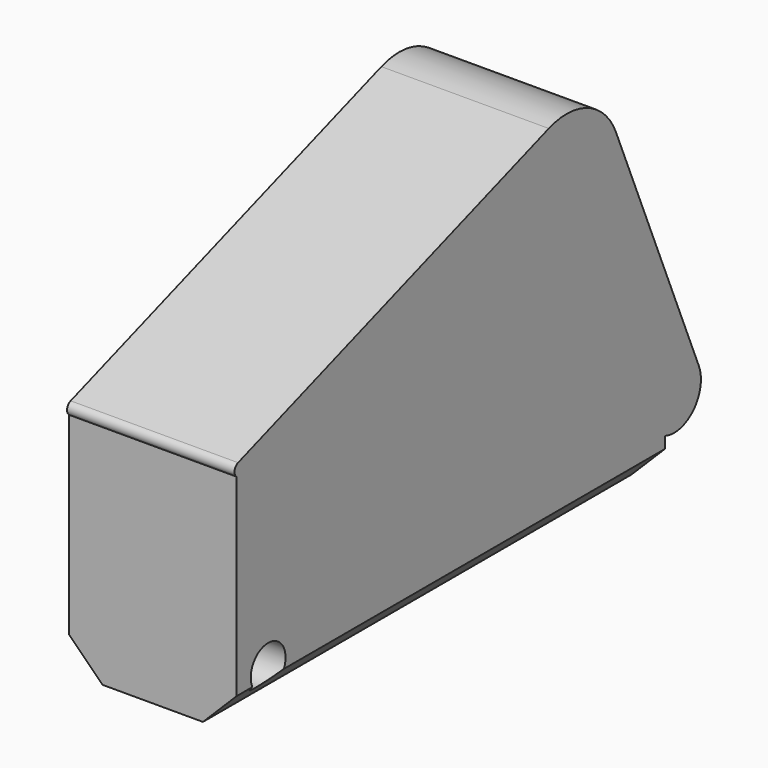
from build123d import *

# Parameters (mm, degrees)
F1_DEPTH     = 25
F3_DEPTH     = 25
F5_D         = 6.5
F6_R         = 10
F7_R         = 5
F8_T1_DEPTH  = 38.943500224
F9_T1_DEPTH  = 105.7168298797
F10_T1_DEPTH = 105.7168298797


# Not quite as in the source:
# - a fillet or chamfer that OpenCascade refuses, or shapes differently, is made with other operations: its cross-section is extruded or revolved along the edge and cut away or added


with BuildPart() as f1:
    # F0 (on Right) → F1 (new body)
    with BuildSketch(Plane.YZ):
        Polygon((-44.8519773781, 0), (35.1480226219, 0), (35.1480226219, 27.3848697543), (-44.8519773781, 35), align=None)
    extrude(amount=F1_DEPTH)

    # F2 (on Right) → F3 (join)
    with BuildSketch(Plane.YZ):
        Polygon((-47.1750815473, 34.6570886492), (45.7401350141, 3.1085526571), (22.3519746214, 59.0625032783), align=None)
    extrude(amount=F3_DEPTH)

    # F5 (through all)
    with Locations(Plane(origin=(0, 0, 0), x_dir=(0, -1, 0), z_dir=(-1, 0, 0))):
        with Locations((38.9309227467, 6.3651315868)):
            Hole(F5_D / 2)

    # F6
    f6_edges = [f1.edges().sort_by_distance(p)[0] for p in [
        (12.5, 22.351975, 59.062503),
    ]]
    fillet(f6_edges, radius=F6_R)

    # F7
    f7_edges = [f1.edges().sort_by_distance(p)[0] for p in [
        (12.5, 45.740135, 3.108553),
    ]]
    fillet(f7_edges, radius=F7_R)

    # F8: fillet of radius 1 on 1 edges, made by hand

    # F8_s2 → F8_t1 (cut)
    with BuildSketch(Plane.YZ.offset(-6.971750112)):
        with BuildLine():
            ThreePointArc((-44.5437819752, 35.580728461), (-45.1967614755, 34.8143003997), (-44.8519773781, 33.8682992754))
            Line((-44.8519773781, 33.8682992754), (-44.8647654465, 33.8529218469))
            ThreePointArc((-44.8647654465, 33.8529218469), (-46.0199597269, 34.2437558604), (-47.1815118114, 34.6381505473))
            Line((-47.1815118114, 34.6381505473), (-47.1817057076, 34.6759598045))
            Line((-47.1817057076, 34.6759598045), (-44.5504061355, 35.5995996162))
            Line((-44.5504061355, 35.5995996162), (-44.5437819752, 35.580728461))
        make_face()
    extrude(amount=F8_T1_DEPTH, mode=Mode.SUBTRACT)

    # F9: chamfer of 5 on 1 edges, made by hand

    # F9_s2 → F9_t1 (cut)
    with BuildSketch(Plane.XZ.offset(-48.0064375617)):
        Polygon((20, 0), (25, 5), (25, 0), align=None)
    extrude(amount=F9_T1_DEPTH, mode=Mode.SUBTRACT)

    # F10: chamfer of 5 on 1 edges, made by hand

    # F10_s2 → F10_t1 (cut)
    with BuildSketch(Plane.XZ.offset(-48.0064375617)):
        Polygon((0, 5), (5, 0), (0, 0), align=None)
    extrude(amount=F10_T1_DEPTH, mode=Mode.SUBTRACT)


solid = f1.part
